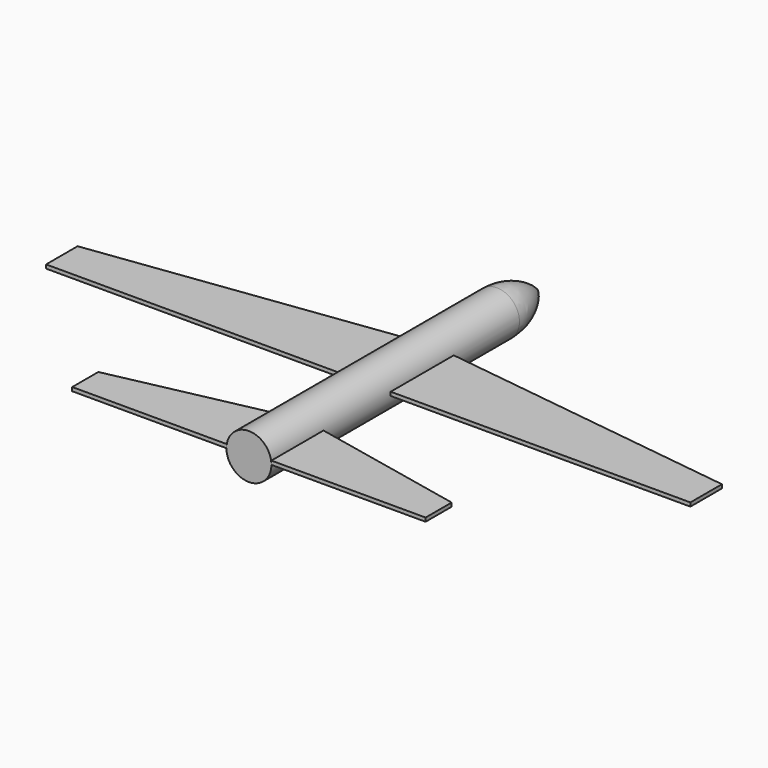
from build123d import *

# Parameters (mm, degrees)
F2_DEPTH = 3.175


# Not quite as in the source:
# - a fillet or chamfer that OpenCascade refuses, or shapes differently, is made with other operations: its cross-section is extruded or revolved along the edge and cut away or added


with BuildPart() as f1:
    # F0 (on Top) → F1 (revolve)
    with BuildSketch(Plane.XY):
        Polygon((0, 55.2100464702), (0, 0), (19.05, 0), (19.05, 304.8), (0, 304.8), (0, 193.2089477777), (0, 126.4116019011), align=None)
    revolve(axis=Axis((19.05, 152.4, 0), (0, 1, 0)))

    # F0 (on Top) → F2 (join)
    with BuildSketch(Plane.XY):
        Polygon((-254, 126.4116019011), (0, 126.4116019011), (0, 193.2089477777), (-254, 159.8102748394), align=None)
        Polygon((38.1, 193.2089477777), (38.1, 126.4116019011), (292.1, 126.4116019011), (292.1, 159.8102748394), align=None)
        Polygon((-130.6934994698, 0), (0, 0), (0, 55.2100464702), (-130.6934994698, 27.6050232351), align=None)
        Polygon((38.1, 55.2100464702), (38.1, 0), (168.7934994698, 0), (168.7934994698, 27.6050232351), align=None)
    extrude(amount=F2_DEPTH)

    # F3: chamfer of 17.78 on 1 edges, made by hand

    # F3_s1 → F3_t2 (revolve, cut)
    with BuildSketch(Plane.XY):
        Polygon((0, 287.02), (17.78, 304.8), (0, 304.8), align=None)
    revolve(axis=Axis((19.05, 304.8, 0), (0, 1, 0)), mode=Mode.SUBTRACT)

    # F4: fillet of radius 58.42 on 1 edges, made by hand

    # F4_s1 → F4_t2 (revolve, cut)
    with BuildSketch(Plane.XY):
        with BuildLine():
            ThreePointArc((0, 262.8216436862), (4.4469577107, 285.1780098049), (17.1108218431, 304.1308218431))
            Line((17.1108218431, 304.1308218431), (0, 287.02))
            Line((0, 287.02), (0, 262.8216436862))
        make_face()
    revolve(axis=Axis((19.05, 287.02, 0), (0, 1, 0)), mode=Mode.SUBTRACT)


solid = f1.part
